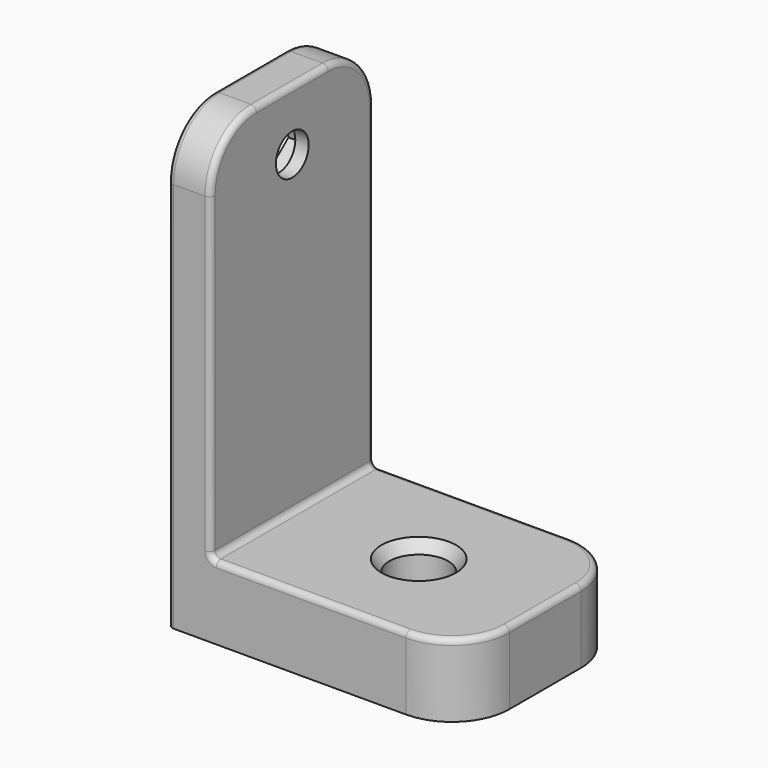
from build123d import *

# Parameters (mm, degrees)
F0_W      = 22
F0_H      = 17.78
F1_DEPTH  = 6.35
F2_W      = 3.7016793489
F2_H      = 17.78
F3_DEPTH  = 39
F6_R      = 2.5527
F8_DEPTH  = 25
F4_R      = 3.2512
F7_R      = 1.524
F10_R     = 1.778
F11_DEPTH = 25
F12_R     = 1.778
F13_DEPTH = 2.54
F14_R     = 5
F15_R     = 0.5


with BuildPart() as f1:
    # F0 (on Top) → F1 (new body)
    with BuildSketch(Plane.XY):
        Rectangle(F0_W, F0_H)
    extrude(amount=F1_DEPTH)

    # F2 (on Top) → F3 (join)
    with BuildSketch(Plane.XY):
        with Locations((-12.8508396745, 0)):
            Rectangle(F2_W, F2_H)
    extrude(amount=F3_DEPTH)

    # F6 (on Top) → F8 (cut)
    with BuildSketch(Plane.XY):
        Circle(F6_R)
    extrude(amount=F8_DEPTH, mode=Mode.SUBTRACT)

    # F4 (on face) → F9 section 0
    with BuildSketch(Plane.XY.offset(6.35)):
        Circle(F4_R)
    # F7 (on offset) → F9 section 1
    with BuildSketch(Plane.XY.offset(3.8862)):
        Circle(F7_R)
    loft(mode=Mode.SUBTRACT)

    # F10 (on face) → F11 (cut)
    with BuildSketch(Plane.YZ.offset(-11)):
        with Locations((0, 33.75)):
            Circle(F10_R)
    extrude(amount=-F11_DEPTH, mode=Mode.SUBTRACT)

    # F12 (on face) → F13 (cut)
    with BuildSketch(Plane(origin=(-14.7016793489, 0, 0), x_dir=(0, -1, 0), z_dir=(-1, 0, 0))):
        Polygon((3.5062095774, 30.91573349), (4.2076515874, 35.36933331), (0.7014420101, 38.20359982), (-3.5062095774, 36.58426651), (-4.2076515874, 32.13066669), (-0.7014420101, 29.29640018), align=None)
        with Locations((0, 33.75)):
            Circle(F12_R, mode=Mode.SUBTRACT)
    extrude(amount=-F13_DEPTH, mode=Mode.SUBTRACT)

    # F14
    f14_edges = [f1.edges().sort_by_distance(p)[0] for p in [
        (11, 8.89, 3.175),
        (11, -8.89, 3.175),
        (-12.85084, 8.89, 39),
        (-12.85084, -8.89, 39),
    ]]
    fillet(f14_edges, radius=F14_R)

    # F15
    f15_edges = [f1.edges().sort_by_distance(p)[0] for p in [
        (-11, -8.89, 20.175),
        (-11, 0, 6.35),
        (-14.701679, -8.89, 17),
        (-14.701679, -7.425534, 37.535534),
        (11, 0, 6.35),
        (9.535534, -7.425534, 6.35),
        (9.535534, 7.425534, 6.35),
        (-2.5, -8.89, 6.35),
        (-2.5, 8.89, 6.35),
        (-11, 8.89, 20.175),
        (-14.701679, 8.89, 17),
        (-14.701679, 7.425534, 37.535534),
        (-14.701679, 0, 39),
        (-11, 7.425534, 37.535534),
        (-11, 0, 39),
        (-11, -7.425534, 37.535534),
    ]]
    fillet(f15_edges, radius=F15_R)


solid = f1.part
